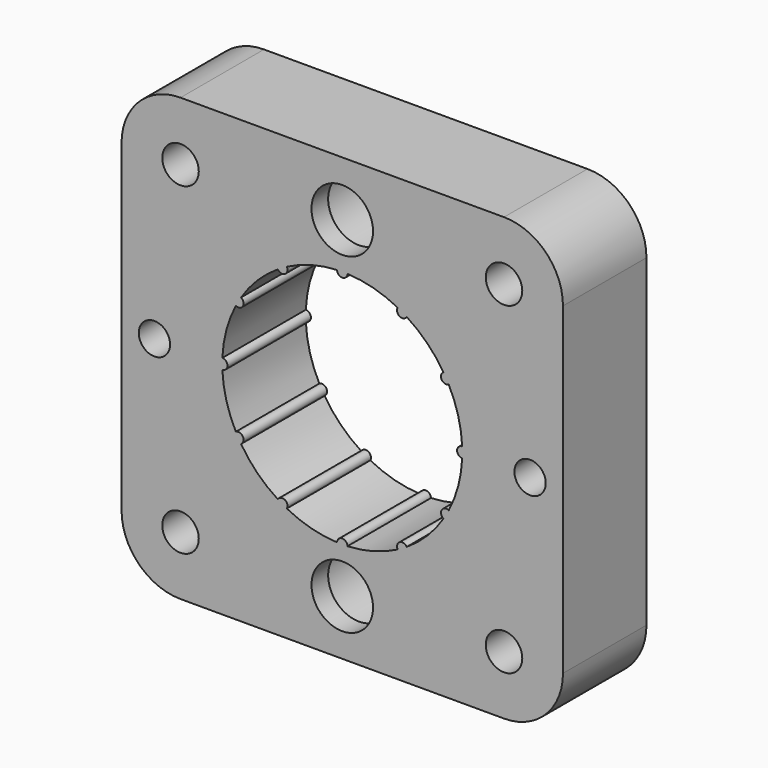
from build123d import *

# Parameters (mm, degrees)
F0_W            = 42.3
F0_H            = 42.3
F0_R            = 1.75
F0_R_2          = 2.95
F0_R_3          = 1.5
F0_R_4          = 11.5
F1_DEPTH        = 10
F2_R            = 3
F3_DEPTH        = 3.5
F4_R            = 4.025
F5_DEPTH        = 8
F6_R            = 5.65
F8_DEPTH        = 10
F8_COPIES_COUNT = 12


# Not quite as in the source:
# - a pattern or mirror of a feature is missing from the dataset's text; its kind, count and spacing are read off the source's solid


with BuildPart() as f1:
    # F0 (on Front) → F1 (new body)
    with BuildSketch(Plane.XZ):
        Rectangle(F0_W, F0_H)
        with Locations((-15.5, -15.5)):
            Circle(F0_R, mode=Mode.SUBTRACT)
        with Locations((0, -15.875)):
            Circle(F0_R_2, mode=Mode.SUBTRACT)
        with Locations((15.5, -15.5)):
            Circle(F0_R, mode=Mode.SUBTRACT)
        with Locations((-18, 0)):
            Circle(F0_R_3, mode=Mode.SUBTRACT)
        with Locations((-15.5, 15.5)):
            Circle(F0_R, mode=Mode.SUBTRACT)
        Circle(F0_R_4, mode=Mode.SUBTRACT)
        with Locations((18, 0)):
            Circle(F0_R_3, mode=Mode.SUBTRACT)
        with Locations((0, 15.875)):
            Circle(F0_R_2, mode=Mode.SUBTRACT)
        with Locations((15.5, 15.5)):
            Circle(F0_R, mode=Mode.SUBTRACT)
    extrude(amount=F1_DEPTH)

    # F2 (on face) → F3 (cut)
    with BuildSketch(Plane(origin=(0, 0, 0), x_dir=(-1, 0, 0), z_dir=(0, 1, 0))):
        with Locations((-15.5, 15.5)):
            Circle(F2_R)
        with Locations((15.5, 15.5)):
            Circle(F2_R)
        with Locations((15.5, -15.5)):
            Circle(F2_R)
        with Locations((-15.5, -15.5)):
            Circle(F2_R)
    extrude(amount=-F3_DEPTH, mode=Mode.SUBTRACT)

    # F4 (on face) → F5 (cut)
    with BuildSketch(Plane(origin=(0, 0, 0), x_dir=(-1, 0, 0), z_dir=(0, 1, 0))):
        with Locations((0, 15.875)):
            Circle(F4_R)
        with Locations((0, -15.875)):
            Circle(F4_R)
    extrude(amount=-F5_DEPTH, mode=Mode.SUBTRACT)

    # F6
    f6_edges = [f1.edges().sort_by_distance(p)[0] for p in [
        (21.15, -5, 21.15),
        (21.15, -5, -21.15),
        (-21.15, -5, 21.15),
        (-21.15, -5, -21.15),
    ]]
    fillet(f6_edges, radius=F6_R)

    # F7 (on face) → F8 (join)
    with BuildSketch(Plane(origin=(0, 0, 0), x_dir=(-1, 0, 0), z_dir=(0, 1, 0))):
        with BuildLine():
            ThreePointArc((11.4891304348, -0.4998818386), (11.5, 0), (11.4891304348, 0.4998818386))
            ThreePointArc((11.4891304348, 0.4998818386), (11, 0), (11.4891304348, -0.4998818386))
        make_face()
    f8 = extrude(amount=-F8_DEPTH)

    # F8_copies: F8 ×12 about axis
    f8_copies_axis = Axis((0, 0, 0), (0, 1, 0))
    for i in range(1, F8_COPIES_COUNT):
        add(f8.rotate(f8_copies_axis, i * 360 / F8_COPIES_COUNT))


solid = f1.part
